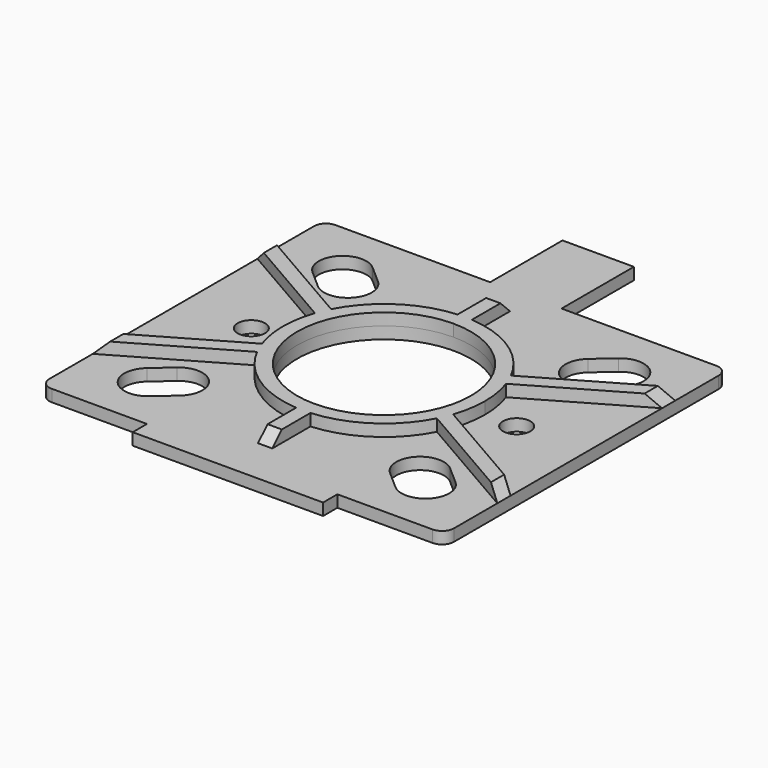
from build123d import *
from build123d import SkipClean  # not in build123d's __all__

# Parameters (mm, degrees)
F0_R     = 1.15
F0_R_2   = 7.3
F0_W     = 16
F0_H     = 1.5
F0_W_2   = 6
F0_H_2   = 7.6
F1_DEPTH = 1
F3_DEPTH = 1
F4_SIZE  = 0.99999


# Not quite as in the source:
# - a fillet or chamfer is up to 0.001 mm smaller than in the source, because OpenCascade refuses the exact size


with BuildPart() as f1:
    # F0 (on Top) → F1 (new body)
    with BuildSketch(Plane.XY):
        with BuildLine():
            Line((8, -14.9), (16, -14.9))
            ThreePointArc((16, -14.9), (16.7071067812, -14.6071067812), (17, -13.9))
            Line((17, -13.9), (17, 13.9))
            ThreePointArc((17, 13.9), (16.7071067812, 14.6071067812), (16, 14.9))
            Line((16, 14.9), (3, 14.9))
            Line((3, 14.9), (-3, 14.9))
            Line((-3, 14.9), (-16, 14.9))
            ThreePointArc((-16, 14.9), (-16.7071067812, 14.6071067812), (-17, 13.9))
            Line((-17, 13.9), (-17, -13.9))
            ThreePointArc((-17, -13.9), (-16.7071067812, -14.6071067812), (-16, -14.9))
            Line((-16, -14.9), (-8, -14.9))
            Line((-8, -14.9), (8, -14.9))
        make_face()
        with BuildLine():
            Line((-8.8286237822, -10.3975032323), (-10.3326805132, -11.71576472))
            ThreePointArc((-10.3326805132, -11.71576472), (-13.1549987319, -11.5299694768), (-12.9692034887, -8.7076512581))
            Line((-12.9692034887, -8.7076512581), (-11.4651467577, -7.3893897703))
            ThreePointArc((-11.4651467577, -7.3893897703), (-8.642828539, -7.5751850136), (-8.8286237822, -10.3975032323))
        make_face(mode=Mode.SUBTRACT)
        with Locations((-11.15, 0)):
            Circle(F0_R, mode=Mode.SUBTRACT)
        with BuildLine():
            ThreePointArc((12.9692034887, -8.7076512581), (13.1549987319, -11.5299694768), (10.3326805132, -11.71576472))
            Line((10.3326805132, -11.71576472), (8.8286237822, -10.3975032323))
            ThreePointArc((8.8286237822, -10.3975032323), (8.642828539, -7.5751850136), (11.4651467577, -7.3893897703))
            Line((11.4651467577, -7.3893897703), (12.9692034887, -8.7076512581))
        make_face(mode=Mode.SUBTRACT)
        Circle(F0_R_2, mode=Mode.SUBTRACT)
        with Locations((11.15, 0)):
            Circle(F0_R, mode=Mode.SUBTRACT)
        with BuildLine():
            Line((-11.4651467577, 7.3893897703), (-12.9692034887, 8.7076512581))
            ThreePointArc((-12.9692034887, 8.7076512581), (-13.1549987319, 11.5299694768), (-10.3326805132, 11.71576472))
            Line((-10.3326805132, 11.71576472), (-8.8286237822, 10.3975032323))
            ThreePointArc((-8.8286237822, 10.3975032323), (-8.642828539, 7.5751850136), (-11.4651467577, 7.3893897703))
        make_face(mode=Mode.SUBTRACT)
        with BuildLine():
            ThreePointArc((10.3326805132, 11.71576472), (13.1549987319, 11.5299694768), (12.9692034887, 8.7076512581))
            Line((12.9692034887, 8.7076512581), (11.4651467577, 7.3893897703))
            ThreePointArc((11.4651467577, 7.3893897703), (8.642828539, 7.5751850136), (8.8286237822, 10.3975032323))
            Line((8.8286237822, 10.3975032323), (10.3326805132, 11.71576472))
        make_face(mode=Mode.SUBTRACT)
        with Locations((0, -15.65)):
            Rectangle(F0_W, F0_H)
        with Locations((0, 18.7)):
            Rectangle(F0_W_2, F0_H_2)
    extrude(amount=F1_DEPTH)

    # F2 (on face) → F3 (join)
    with BuildSketch(Plane.XY.offset(1)):
        with BuildLine():
            ThreePointArc((0, 7.3), (5.1618795027, 5.1618795027), (7.3, 0))
            ThreePointArc((7.3, 0), (5.1618795027, -5.1618795027), (0, -7.3))
            Line((0, -7.3), (0.6, -7.3))
            Line((0.6, -7.3), (0.6, -8.4787970845))
            ThreePointArc((0.6, -8.4787970845), (4.6794449698, -7.0959703195), (7.5571902637, -3.8908707661))
            ThreePointArc((7.5571902637, -3.8908707661), (7.8146834893, -3.3437586578), (8.0326290711, -2.7797248435))
            ThreePointArc((8.0326290711, -2.7797248435), (8.3823429632, -1.4093709404), (8.5, 0))
            ThreePointArc((8.5, 0), (8.3823429632, 1.4093709404), (8.0326290711, 2.7797248435))
            ThreePointArc((8.0326290711, 2.7797248435), (7.8146834893, 3.3437586578), (7.5571902637, 3.8908707661))
            ThreePointArc((7.5571902637, 3.8908707661), (4.6794449698, 7.0959703195), (0.6, 8.4787970845))
            Line((0.6, 8.4787970845), (0.6, 7.3))
            Line((0.6, 7.3), (0, 7.3))
        make_face()
        with BuildLine():
            Line((-0.6, 7.3), (0, 7.3))
            Line((0, 7.3), (0.6, 7.3))
            Line((0.6, 7.3), (0.6, 8.4787970845))
            ThreePointArc((0.6, 8.4787970845), (0, 8.5), (-0.6, 8.4787970845))
            Line((-0.6, 8.4787970845), (-0.6, 7.3))
        make_face()
        with BuildLine():
            ThreePointArc((0, -7.3), (-7.3, 0), (0, 7.3))
            Line((0, 7.3), (-0.6, 7.3))
            Line((-0.6, 7.3), (-0.6, 8.4787970845))
            ThreePointArc((-0.6, 8.4787970845), (-4.6794449698, 7.0959703195), (-7.5571902637, 3.8908707661))
            ThreePointArc((-7.5571902637, 3.8908707661), (-7.8146834893, 3.3437586578), (-8.0326290711, 2.7797248435))
            ThreePointArc((-8.0326290711, 2.7797248435), (-8.5, 0), (-8.0326290711, -2.7797248435))
            ThreePointArc((-8.0326290711, -2.7797248435), (-7.8146834893, -3.3437586578), (-7.5571902637, -3.8908707661))
            ThreePointArc((-7.5571902637, -3.8908707661), (-4.6794449698, -7.0959703195), (-0.6, -8.4787970845))
            Line((-0.6, -8.4787970845), (-0.6, -7.3))
            Line((-0.6, -7.3), (0, -7.3))
        make_face()
        with BuildLine():
            Line((0.6, -7.3), (0, -7.3))
            Line((0, -7.3), (-0.6, -7.3))
            Line((-0.6, -7.3), (-0.6, -8.4787970845))
            ThreePointArc((-0.6, -8.4787970845), (0, -8.5), (0.6, -8.4787970845))
            Line((0.6, -8.4787970845), (0.6, -7.3))
        make_face()
        with BuildLine():
            ThreePointArc((-0.6, 8.4787970845), (0, 8.5), (0.6, 8.4787970845))
            Line((0.6, 8.4787970845), (0.6, 11.4843371598))
            Line((0.6, 11.4843371598), (-0.6, 11.4843371598))
            Line((-0.6, 11.4843371598), (-0.6, 8.4787970845))
        make_face()
        with BuildLine():
            Line((0.6, -11.4843371598), (0.6, -8.4787970845))
            ThreePointArc((0.6, -8.4787970845), (0, -8.5), (-0.6, -8.4787970845))
            Line((-0.6, -8.4787970845), (-0.6, -11.4843371598))
            Line((-0.6, -11.4843371598), (0.6, -11.4843371598))
        make_face()
        with BuildLine():
            ThreePointArc((-8.0326290711, 2.7797248435), (-7.8146834893, 3.3437586578), (-7.5571902637, 3.8908707661))
            Line((-7.5571902637, 3.8908707661), (-17, 9.3426795092))
            Line((-17, 9.3426795092), (-17, 7.9570388632))
            Line((-17, 7.9570388632), (-8.0326290711, 2.7797248435))
        make_face()
        with BuildLine():
            Line((-17, -9.3426795092), (-7.5571902637, -3.8908707661))
            ThreePointArc((-7.5571902637, -3.8908707661), (-7.8146834893, -3.3437586578), (-8.0326290711, -2.7797248435))
            Line((-8.0326290711, -2.7797248435), (-17, -7.9570388632))
            Line((-17, -7.9570388632), (-17, -9.3426795092))
        make_face()
        with BuildLine():
            ThreePointArc((8.0326290711, -2.7797248435), (7.8146834893, -3.3437586578), (7.5571902637, -3.8908707661))
            Line((7.5571902637, -3.8908707661), (17, -9.3426795092))
            Line((17, -9.3426795092), (17, -7.9570388632))
            Line((17, -7.9570388632), (8.0326290711, -2.7797248435))
        make_face()
        with BuildLine():
            Line((17, 9.3426795092), (7.5571902637, 3.8908707661))
            ThreePointArc((7.5571902637, 3.8908707661), (7.8146834893, 3.3437586578), (8.0326290711, 2.7797248435))
            Line((8.0326290711, 2.7797248435), (17, 7.9570388632))
            Line((17, 7.9570388632), (17, 9.3426795092))
        make_face()
    with SkipClean():  # cleaning this boolean's faces spoils the solid; the shape is the same uncleaned
        extrude(amount=F3_DEPTH)

    # F4 (size 1 in the source; OpenCascade refuses exactly that, so slightly less here)
    f4_edges = [f1.edges().sort_by_distance(p)[0] for p in [
        (0, 11.484337, 1),
        (0, -11.484337, 1),
        (-17, -8.649859, 2),
        (17, -8.649859, 2),
        (-17, 8.649859, 2),
        (17, 8.649859, 2),
    ]]
    chamfer(f4_edges, length=F4_SIZE)


solid = f1.part
